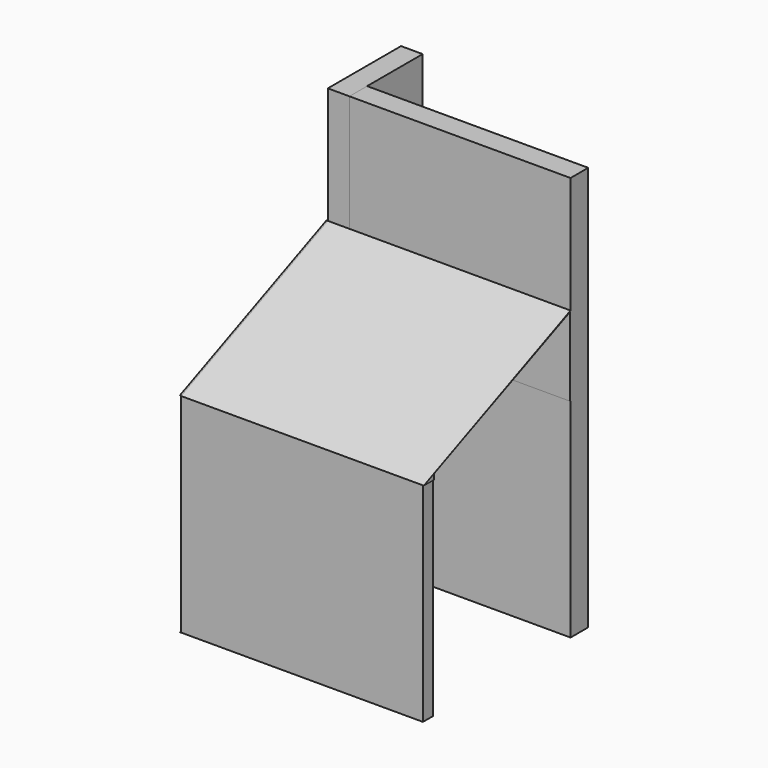
from build123d import *

# Parameters (mm, degrees)
F1_DEPTH  = 1800
F4_DEPTH  = 10
F3_W      = 198.5935460704
F3_H      = 125.2263307571
F3_H_2    = 119
F3_W_2    = 305
F6_DEPTH  = 10
F7_DEPTH  = 1806.4861297607
F9_DEPTH  = 2295.1808217913
F11_DEPTH = 1985.6109861284
F12_W     = 719.2032337189
F12_H     = 3839.0393257141
F13_DEPTH = 2175.1913074404
F14_DEPTH = 160.8089450747
F15_W     = 1610
F15_H     = 74.8850554228
F16_DEPTH = 2483.9819669724


with BuildPart() as f1:
    # F0 (on Right) → F1 (new body)
    with BuildSketch(Plane.YZ):
        Polygon((-95, -290.000010696), (0, -290.000010696), (0, 1299.999989304), (-95, 1259.999989304), align=None)
    extrude(amount=F1_DEPTH)

    # F15 (on face) → F16 (cut)
    with BuildSketch(Plane(origin=(0, 0, -290.000010696), x_dir=(1, 0, 0), z_dir=(0, 0, -1))):
        with Locations((900, 37.4425277114)):
            Rectangle(F15_W, F15_H)
    extrude(amount=-F16_DEPTH, mode=Mode.SUBTRACT)


with BuildPart() as f4:
    # F2 (on face) → F4 (new body)
    with BuildSketch(Plane(origin=(0, 0, 0), x_dir=(0, -1, 0), z_dir=(-1, 0, 0))):
        Polygon((-1270, 1852.8258800507), (-1270, 1259.999989304), (0, 1259.999989304), (0, 1299.999989304), (95, 1259.999989304), align=None)
    extrude(amount=F4_DEPTH)

    # F5 (on face) → F6 (join)
    with BuildSketch(Plane(origin=(-10, 0, 0), x_dir=(0, -1, 0), z_dir=(-1, 0, 0))):
        Polygon((-305.2440285683, 1259.999989304), (-305.2440285683, 1137.7295255661), (0, 1138.8988494873), (0, 1259.999989304), align=None)
    extrude(amount=-F6_DEPTH)


with BuildPart() as f4b:
    # F3 (on face) → F4, piece 2 (new body)
    with BuildSketch(Plane(origin=(0, 0, 0), x_dir=(0, -1, 0), z_dir=(-1, 0, 0))):
        with Locations((-1169.9069863149, 1200.3113059998)):
            Rectangle(F3_W, F3_H)
        with Locations((-1169.9069863149, 840.1981406212)):
            Rectangle(F3_W, F3_H_2)
        with Locations((-1169.9069863149, 1078.1981406212)):
            Rectangle(F3_W, F3_H_2)
        with Locations((-1169.9069863149, 959.1981406212)):
            Rectangle(F3_W, F3_H_2)
        with Locations((-1169.9069863149, 602.1981406212)):
            Rectangle(F3_W, F3_H_2)
        with Locations((-1169.9069863149, 721.1981406212)):
            Rectangle(F3_W, F3_H_2)
        with Locations((-1169.9069863149, 483.1981406212)):
            Rectangle(F3_W, F3_H_2)
        with Locations((-1169.9069863149, 364.1981406212)):
            Rectangle(F3_W, F3_H_2)
        with Locations((-1169.9069863149, 245.1981406212)):
            Rectangle(F3_W, F3_H_2)
        with Locations((-1169.9069863149, 126.1981406212)):
            Rectangle(F3_W, F3_H_2)
        Polygon((-1070.6102132797, 66.6981406212), (-1269.2037593501, 66.6981406212), (-1269.2037593501, 0), (-1269.4583772772, -52.3018593788), (-1070.6102132797, -52.3018593788), align=None)
        Polygon((-1070.6102132797, -171.3018593788), (-1070.6102132797, -52.3018593788), (-1269.4583772772, -52.3018593788), (-1270.0376976624, -171.3018593788), align=None)
        Polygon((-1070.6102132797, -288.9040708542), (-1070.6102132797, -171.3018593788), (-1270.0376976624, -171.3018593788), (-1270.6102132797, -288.9040708542), align=None)
    extrude(amount=F4_DEPTH)


with BuildPart() as f4c:
    # F3 (on face) → F4, piece 3 (new body)
    with BuildSketch(Plane(origin=(0, 0, 0), x_dir=(0, -1, 0), z_dir=(-1, 0, 0))):
        Polygon((0, -171.3018593788), (-305, -171.3018593788), (-305, -290.3018593788), (95, -290.3018593788), (95, -290.000010696), (0, -290.000010696), align=None)
        with Locations((-152.5, -111.8018593788)):
            Rectangle(F3_W_2, F3_H_2)
        with Locations((-152.5, 7.1981406212)):
            Rectangle(F3_W_2, F3_H_2)
        with Locations((-152.5, 126.1981406212)):
            Rectangle(F3_W_2, F3_H_2)
        with Locations((-152.5, 245.1981406212)):
            Rectangle(F3_W_2, F3_H_2)
        with Locations((-152.5, 364.1981406212)):
            Rectangle(F3_W_2, F3_H_2)
        with Locations((-152.5, 483.1981406212)):
            Rectangle(F3_W_2, F3_H_2)
        with Locations((-152.5, 602.1981406212)):
            Rectangle(F3_W_2, F3_H_2)
        with Locations((-152.5, 840.1981406212)):
            Rectangle(F3_W_2, F3_H_2)
        with Locations((-152.5, 959.1981406212)):
            Rectangle(F3_W_2, F3_H_2)
        with Locations((-152.5, 721.1981406212)):
            Rectangle(F3_W_2, F3_H_2)
        with Locations((-152.5, 1078.1981406212)):
            Rectangle(F3_W_2, F3_H_2)
    extrude(amount=F4_DEPTH)


with BuildPart() as f7:
    # F2 (on face) → F7 (new body)
    with BuildSketch(Plane(origin=(0, 0, 0), x_dir=(0, -1, 0), z_dir=(-1, 0, 0))):
        Polygon((-1951.2008428574, -290.000010696), (-1270, -290.000010696), (-1270, 1259.999989304), (-1270, 1852.8258800507), (-1270, 2720.9904193878), (-1951.2008428574, 2720.9904193878), align=None)
        Polygon((-1270, 1852.8258800507), (-1270, 1259.999989304), (0, 1259.999989304), (95, 1259.999989304), align=None)
    extrude(amount=-F7_DEPTH)

    # F8 (on face) → F9 (cut)
    with BuildSketch(Plane.YZ.offset(1806.4861297607)):
        Polygon((305.9136271477, 1261.8664503098), (305.9136271477, 1258.1008672714), (379.9477815628, 1258.1008672714), (522.2533345222, 1258.1008672714), (570.3758001328, 1258.1008672714), (747.250020504, 1258.1008672714), (916.7550802231, 1258.1008672714), (1097.1890687943, 1258.1008672714), (1266.1670446396, 1258.1008672714), (1266.1670446396, 1261.8664503098), (1266.1670446396, 1289.4487380981), (1266.1670446396, 1648.1994390488), (1266.1670446396, 1803.9075136185), (1266.1670446396, 1846.3387489319), (305.9136271477, 1433.1557750702), align=None)
        Polygon((305.9136271477, 1261.8664503098), (305.9136271477, 1259.999989304), (1266.1670446396, 1259.999989304), (1266.1670446396, 1261.8664503098), (1266.1670446396, 1289.4487380981), (1266.1670446396, 1648.1994390488), (1266.1670446396, 1803.9075136185), (1266.1670446396, 1846.3387489319), (305.9136271477, 1433.1557750702), align=None)
    extrude(amount=-F9_DEPTH, mode=Mode.SUBTRACT)

    # F10 (on face) → F11 (cut)
    with BuildSketch(Plane.YZ.offset(1806.4861297607)):
        Polygon((305.9136271477, 1259.999989304), (305.9136271477, 1433.1557750702), (202.2104150255, 1388.116984521), (8.5436779362, 1304.0066138815), (0.8936976359, 1300.6841916209), (0.8936976359, 1259.999989304), align=None)
    extrude(amount=-F11_DEPTH, mode=Mode.SUBTRACT)

    # F12 (on face) → F13 (cut)
    with BuildSketch(Plane(origin=(0, 0, 0), x_dir=(0, -1, 0), z_dir=(-1, 0, 0))):
        with Locations((-1794.2711114883, 1262.0453834534)):
            Rectangle(F12_W, F12_H)
    extrude(amount=-F13_DEPTH, mode=Mode.SUBTRACT)


with BuildPart() as f14:
    # F2 (on face) → F14 (new body)
    with BuildSketch(Plane(origin=(0, 0, 0), x_dir=(0, -1, 0), z_dir=(-1, 0, 0))):
        Polygon((-1951.2008428574, -290.000010696), (-1270, -290.000010696), (-1270, 1259.999989304), (-1270, 1852.8258800507), (-1270, 2720.9904193878), (-1951.2008428574, 2720.9904193878), align=None)
    extrude(amount=-F14_DEPTH)


solid = Compound([f1.part, f4.part, f4b.part, f4c.part, f7.part, f14.part])
